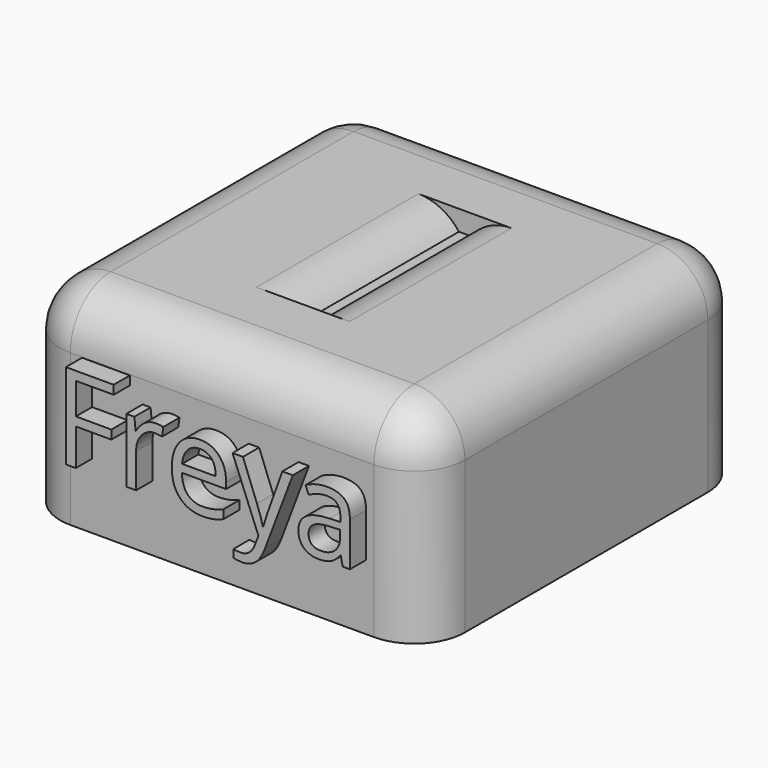
from build123d import *

# Parameters (mm, degrees)
F0_W         = 40
F0_H         = 40
F0_W_2       = 1.2
F0_H_2       = 20
F1_DEPTH     = 20
F2_DEPTH     = 2
F3_T1_DEPTH  = 20
F3_T3_DEPTH  = 27.5
F3_T5_DEPTH  = 30
F3_T7_DEPTH  = 30
F3_S11_W     = 5.1
F3_S11_H     = 5.1
F3_T12_DEPTH = 5.1
F3_S17_W     = 5.1
F3_S17_H     = 5.1
F3_T18_DEPTH = 5.1
F3_S23_W     = 5.1
F3_S23_H     = 5.1
F3_T24_DEPTH = 5.1
F3_S29_W     = 5.1
F3_S29_H     = 5.1
F3_T30_DEPTH = 5.1
F4_TEXT_SIZE = 11.8606375093
F5_DEPTH     = 2


# Not quite as in the source:
# - a fillet or chamfer that OpenCascade refuses, or shapes differently, is made with other operations: its cross-section is extruded or revolved along the edge and cut away or added
# - Text() gives the source's letters only with a copy of the font that has no kerning and outlines rounded to 1/6400 em; it was checked with that copy


with BuildPart() as f1:
    # F0 (on Top) → F1 (new body)
    with BuildSketch(Plane.XY):
        Rectangle(F0_W, F0_H)
        Rectangle(F0_W_2, F0_H_2, mode=Mode.SUBTRACT)
        Rectangle(F0_W_2, F0_H_2)
    extrude(amount=-F1_DEPTH)

    # F0 (on Top) → F2 (cut)
    with BuildSketch(Plane.XY):
        Rectangle(F0_W_2, F0_H_2)
    extrude(amount=-F2_DEPTH, mode=Mode.SUBTRACT)

    # F3: fillet of radius 5 on 10 edges, made by hand

    # F3_s2 → F3_t1 (cut)
    with BuildSketch(Plane.XZ.offset(-10)):
        with BuildLine():
            ThreePointArc((4.6, 0), (2.3639320225, -0.527864045), (0.6, -2))
            Line((0.6, -2), (0.6, 0))
            Line((0.6, 0), (4.6, 0))
        make_face()
        with BuildLine():
            ThreePointArc((-4.6, 0), (-2.3639320225, -0.527864045), (-0.6, -2))
            Line((-0.6, -2), (-0.6, 0))
            Line((-0.6, 0), (-4.6, 0))
        make_face()
    extrude(amount=F3_T1_DEPTH, mode=Mode.SUBTRACT)

    # F3_s4 → F3_t3 (cut)
    with BuildSketch(Plane.XY.offset(-32.5)):
        with BuildLine():
            ThreePointArc((15, -20), (18.5355339059, -18.5355339059), (20, -15))
            Line((20, -15), (20, -20))
            Line((20, -20), (15, -20))
        make_face()
        with BuildLine():
            ThreePointArc((20, 15), (18.5355339059, 18.5355339059), (15, 20))
            Line((15, 20), (20, 20))
            Line((20, 20), (20, 15))
        make_face()
        with BuildLine():
            ThreePointArc((-15, -20), (-18.5355339059, -18.5355339059), (-20, -15))
            Line((-20, -15), (-20, -20))
            Line((-20, -20), (-15, -20))
        make_face()
        with BuildLine():
            ThreePointArc((-20, 15), (-18.5355339059, 18.5355339059), (-15, 20))
            Line((-15, 20), (-20, 20))
            Line((-20, 20), (-20, 15))
        make_face()
    extrude(amount=F3_T3_DEPTH, mode=Mode.SUBTRACT)

    # F3_s6 → F3_t5 (cut)
    with BuildSketch(Plane.XZ.offset(-15)):
        with BuildLine():
            ThreePointArc((20, -5), (18.5355339059, -1.4644660941), (15, 0))
            Line((15, 0), (20, 0))
            Line((20, 0), (20, -5))
        make_face()
        with BuildLine():
            ThreePointArc((-20, -5), (-18.5355339059, -1.4644660941), (-15, 0))
            Line((-15, 0), (-20, 0))
            Line((-20, 0), (-20, -5))
        make_face()
    extrude(amount=F3_T5_DEPTH, mode=Mode.SUBTRACT)

    # F3_s8 → F3_t7 (cut)
    with BuildSketch(Plane.YZ.offset(-15)):
        with BuildLine():
            ThreePointArc((15, 0), (18.5355339059, -1.4644660941), (20, -5))
            Line((20, -5), (20, 0))
            Line((20, 0), (15, 0))
        make_face()
        with BuildLine():
            ThreePointArc((-20, -5), (-18.5355339059, -1.4644660941), (-15, 0))
            Line((-15, 0), (-20, 0))
            Line((-20, 0), (-20, -5))
        make_face()
    extrude(amount=F3_T7_DEPTH, mode=Mode.SUBTRACT)


with BuildPart() as f3_tool10:
    # F3_s11 → F3_t12 (new body)
    with BuildSketch(Plane.XZ.offset(15)):
        with Locations((17.55, -2.45)):
            Rectangle(F3_S11_W, F3_S11_H)
    extrude(amount=F3_T12_DEPTH)

    # F3_s13 → F3_t14 (revolve, cut)
    with BuildSketch(Plane(origin=(15, -15, -5), x_dir=(-0.7071067812, 0, -0.7071067812), z_dir=(-0.7071067812, 0, 0.7071067812))):
        with BuildLine():
            ThreePointArc((0, -5), (5, 0), (0, 5))
            Line((0, 5), (0, -5))
        make_face()
    revolve(axis=Axis((15, -15, -5), (0, -1, 0)), mode=Mode.SUBTRACT)


with BuildPart() as f1_1:
    add(f1.part)

    # F3_t9: cut F3_tool10
    add(f3_tool10.part, mode=Mode.SUBTRACT)


with BuildPart() as f3_tool16:
    # F3_s17 → F3_t18 (new body)
    with BuildSketch(Plane.YZ.offset(15)):
        with Locations((17.55, -2.45)):
            Rectangle(F3_S17_W, F3_S17_H)
    extrude(amount=F3_T18_DEPTH)

    # F3_s19 → F3_t20 (revolve, cut)
    with BuildSketch(Plane(origin=(15, 15, -5), x_dir=(0, -0.7071067812, -0.7071067812), z_dir=(0, -0.7071067812, 0.7071067812))):
        with BuildLine():
            ThreePointArc((0, -5), (5, 0), (0, 5))
            Line((0, 5), (0, -5))
        make_face()
    revolve(axis=Axis((15, 15, -5), (1, 0, 0)), mode=Mode.SUBTRACT)


with BuildPart() as f1_2:
    add(f1_1.part)

    # F3_t15: cut F3_tool16
    add(f3_tool16.part, mode=Mode.SUBTRACT)


with BuildPart() as f3_tool22:
    # F3_s23 → F3_t24 (new body)
    with BuildSketch(Plane.XZ.offset(15)):
        with Locations((-17.55, -2.45)):
            Rectangle(F3_S23_W, F3_S23_H)
    extrude(amount=F3_T24_DEPTH)

    # F3_s25 → F3_t26 (revolve, cut)
    with BuildSketch(Plane(origin=(-15, -15, -5), x_dir=(0.7071067812, 0, -0.7071067812), z_dir=(-0.7071067812, 0, -0.7071067812))):
        with BuildLine():
            ThreePointArc((0, -5), (5, 0), (0, 5))
            Line((0, 5), (0, -5))
        make_face()
    revolve(axis=Axis((-15, -15, -5), (0, -1, 0)), mode=Mode.SUBTRACT)


with BuildPart() as f1_3:
    add(f1_2.part)

    # F3_t21: cut F3_tool22
    add(f3_tool22.part, mode=Mode.SUBTRACT)


with BuildPart() as f3_tool28:
    # F3_s29 → F3_t30 (new body)
    with BuildSketch(Plane.YZ.offset(-15)):
        with Locations((17.55, -2.45)):
            Rectangle(F3_S29_W, F3_S29_H)
    extrude(amount=-F3_T30_DEPTH)

    # F3_s31 → F3_t32 (revolve, cut)
    with BuildSketch(Plane(origin=(-15, 15, -5), x_dir=(0, -0.7071067812, -0.7071067812), z_dir=(0, 0.7071067812, -0.7071067812))):
        with BuildLine():
            ThreePointArc((0, -5), (5, 0), (0, 5))
            Line((0, 5), (0, -5))
        make_face()
    revolve(axis=Axis((-15, 15, -5), (-1, 0, 0)), mode=Mode.SUBTRACT)


with BuildPart() as f1_4:
    add(f1_3.part)

    # F3_t27: cut F3_tool28
    add(f3_tool28.part, mode=Mode.SUBTRACT)

    # F4 (on face) → F5 (join)
    with BuildSketch(Plane.XZ.offset(20)):
        with Locations((-15, -13.5396590067)):
            Text('Freya', F4_TEXT_SIZE, font='Open Sans', text_align=(TextAlign.LEFT, TextAlign.BOTTOM))
    extrude(amount=F5_DEPTH)


solid = f1_4.part
